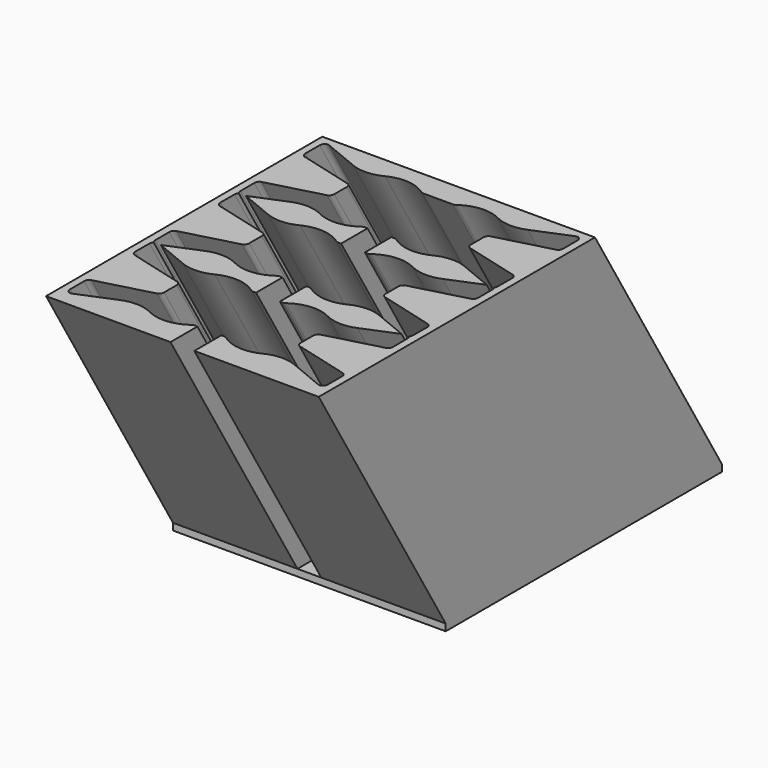
from build123d import *

# Parameters (mm, degrees)
F1_DEPTH  = 88.9
F3_W      = 40.64
F3_H      = 44.1143267043
F4_DEPTH  = 12.7
F9_ANGLE  = -59
F11_W     = 127.9208920896
F11_H     = 131.2496848404
F11_W_2   = 76.2
F11_H_2   = 39.37
F12_DEPTH = 76.2
F14_DEPTH = 1.016


with BuildPart() as f1:
    # F0 (on Front) → F1 (new body)
    with BuildSketch(Plane.XZ):
        with BuildLine():
            Line((-2.2330590469, 18.2673970938), (-1.778, 18.2673970938))
            Line((-1.778, 18.2673970938), (-1.778, 22.4996029062))
            Line((-1.778, 22.4996029062), (-2.2330590469, 22.4996029062))
            ThreePointArc((-2.2330590469, 22.4996029062), (-2.4055915324, 22.4757146321), (-2.5651429052, 22.4058471312))
            ThreePointArc((-2.5651429052, 22.4058471312), (-5.4252105459, 21.4850287563), (-8.3884412084, 21.9821780602))
            ThreePointArc((-8.3884412084, 21.9821780602), (-10.6860377447, 22.4927612394), (-13.0117790963, 22.1314134961))
            Line((-13.0117790963, 22.1314134961), (-17.9445793555, 20.3835))
            Line((-17.9445793555, 20.3835), (-13.0117790963, 18.6355865039))
            ThreePointArc((-13.0117790963, 18.6355865039), (-10.6860377447, 18.2742387606), (-8.3884412084, 18.7848219398))
            ThreePointArc((-8.3884412084, 18.7848219398), (-5.4252105459, 19.2819712437), (-2.5651429052, 18.3611528688))
            ThreePointArc((-2.5651429052, 18.3611528688), (-2.4055915324, 18.2912853679), (-2.2330590469, 18.2673970938))
        make_face()
    extrude(amount=F1_DEPTH)


with BuildPart() as f1b:
    # F0 (on Front) → F1, piece 2 (new body)
    with BuildSketch(Plane.XZ):
        with BuildLine():
            Line((13.0117790963, 18.6355865039), (17.9445793555, 20.3835))
            Line((17.9445793555, 20.3835), (13.0117790963, 22.1314134961))
            ThreePointArc((13.0117790963, 22.1314134961), (10.6860377447, 22.4927612394), (8.3884412084, 21.9821780602))
            ThreePointArc((8.3884412084, 21.9821780602), (5.4252105459, 21.4850287563), (2.5651429052, 22.4058471312))
            ThreePointArc((2.5651429052, 22.4058471312), (2.4055915324, 22.4757146321), (2.2330590469, 22.4996029062))
            Line((2.2330590469, 22.4996029062), (1.778, 22.4996029062))
            Line((1.778, 22.4996029062), (1.778, 18.2673970938))
            Line((1.778, 18.2673970938), (2.2330590469, 18.2673970938))
            ThreePointArc((2.2330590469, 18.2673970938), (2.4055915324, 18.2912853679), (2.5651429052, 18.3611528688))
            ThreePointArc((2.5651429052, 18.3611528688), (5.4252105459, 19.2819712437), (8.3884412084, 18.7848219398))
            ThreePointArc((8.3884412084, 18.7848219398), (10.6860377447, 18.2742387606), (13.0117790963, 18.6355865039))
        make_face()
    extrude(amount=F1_DEPTH)


with BuildPart() as f1c:
    # F0 (on Front) → F1, piece 3 (new body)
    with BuildSketch(Plane.XZ):
        with BuildLine():
            Line((13.0117790963, 5.0465865039), (17.9445793555, 6.7945))
            Line((17.9445793555, 6.7945), (13.0117790963, 8.5424134961))
            ThreePointArc((13.0117790963, 8.5424134961), (10.6860377447, 8.9037612394), (8.3884412084, 8.3931780602))
            ThreePointArc((8.3884412084, 8.3931780602), (5.4252105459, 7.8960287563), (2.5651429052, 8.8168471312))
            ThreePointArc((2.5651429052, 8.8168471312), (2.4055915324, 8.8867146321), (2.2330590469, 8.9106029062))
            Line((2.2330590469, 8.9106029062), (1.778, 8.9106029062))
            Line((1.778, 8.9106029062), (1.778, 4.6783970938))
            Line((1.778, 4.6783970938), (2.2330590469, 4.6783970938))
            ThreePointArc((2.2330590469, 4.6783970938), (2.4055915324, 4.7022853679), (2.5651429052, 4.7721528688))
            ThreePointArc((2.5651429052, 4.7721528688), (5.4252105459, 5.6929712437), (8.3884412084, 5.1958219398))
            ThreePointArc((8.3884412084, 5.1958219398), (10.6860377447, 4.6852387606), (13.0117790963, 5.0465865039))
        make_face()
    extrude(amount=F1_DEPTH)


with BuildPart() as f1d:
    # F0 (on Front) → F1, piece 4 (new body)
    with BuildSketch(Plane.XZ):
        with BuildLine():
            Line((-2.2330590469, 4.6783970938), (-1.778, 4.6783970938))
            Line((-1.778, 4.6783970938), (-1.778, 8.9106029062))
            Line((-1.778, 8.9106029062), (-2.2330590469, 8.9106029062))
            ThreePointArc((-2.2330590469, 8.9106029062), (-2.4055915324, 8.8867146321), (-2.5651429052, 8.8168471312))
            ThreePointArc((-2.5651429052, 8.8168471312), (-5.4252105459, 7.8960287563), (-8.3884412084, 8.3931780602))
            ThreePointArc((-8.3884412084, 8.3931780602), (-10.6860377447, 8.9037612394), (-13.0117790963, 8.5424134961))
            Line((-13.0117790963, 8.5424134961), (-17.9445793555, 6.7945))
            Line((-17.9445793555, 6.7945), (-13.0117790963, 5.0465865039))
            ThreePointArc((-13.0117790963, 5.0465865039), (-10.6860377447, 4.6852387606), (-8.3884412084, 5.1958219398))
            ThreePointArc((-8.3884412084, 5.1958219398), (-5.4252105459, 5.6929712437), (-2.5651429052, 4.7721528688))
            ThreePointArc((-2.5651429052, 4.7721528688), (-2.4055915324, 4.7022853679), (-2.2330590469, 4.6783970938))
        make_face()
    extrude(amount=F1_DEPTH)


with BuildPart() as f1e:
    # F0 (on Front) → F1, piece 5 (new body)
    with BuildSketch(Plane.XZ):
        with BuildLine():
            ThreePointArc((10.6693075207, 1.6245687681), (10.3142300694, 1.4013840597), (10.1757328957, 1.0055179921))
            Line((10.1757328957, 1.0055179921), (10.1757328957, 0))
            Line((10.1757328957, 0), (10.1757328957, -1.0055179921))
            ThreePointArc((10.1757328957, -1.0055179921), (10.3142300694, -1.4013840597), (10.6693075207, -1.6245687681))
            Line((10.6693075207, -1.6245687681), (18.7232144628, -3.4645257695))
            ThreePointArc((18.7232144628, -3.4645257695), (19.0794060399, -3.6891118844), (19.2167789926, -4.0871571512))
            Line((19.2167789926, -4.0871571512), (19.2040435859, -6.3456730598))
            ThreePointArc((19.2040435859, -6.3456730598), (18.9340250914, -6.8617277779), (18.3569658643, -6.9406271299))
            Line((18.3569658643, -6.9406271299), (13.0117790963, -5.0465865039))
            ThreePointArc((13.0117790963, -5.0465865039), (10.6860377447, -4.6852387606), (8.3884412084, -5.1958219398))
            ThreePointArc((8.3884412084, -5.1958219398), (5.4252105459, -5.6929712437), (2.5651429052, -4.7721528688))
            ThreePointArc((2.5651429052, -4.7721528688), (2.4055915324, -4.7022853679), (2.2330590469, -4.6783970938))
            Line((2.2330590469, -4.6783970938), (1.778, -4.6783970938))
            Line((1.778, -4.6783970938), (1.778, -8.9796995744))
            Line((1.778, -8.9796995744), (20.32, -8.9796995744))
            Line((20.32, -8.9796995744), (20.32, 35.1346271299))
            Line((20.32, 35.1346271299), (-20.32, 35.1346271299))
            Line((-20.32, 35.1346271299), (-20.32, -8.9796995744))
            Line((-20.32, -8.9796995744), (-1.778, -8.9796995744))
            Line((-1.778, -8.9796995744), (-1.778, -4.6783970938))
            Line((-1.778, -4.6783970938), (-2.2330590469, -4.6783970938))
            ThreePointArc((-2.2330590469, -4.6783970938), (-2.4055915324, -4.7022853679), (-2.5651429052, -4.7721528688))
            ThreePointArc((-2.5651429052, -4.7721528688), (-5.4252105459, -5.6929712437), (-8.3884412084, -5.1958219398))
            ThreePointArc((-8.3884412084, -5.1958219398), (-10.6860377447, -4.6852387606), (-13.0117790963, -5.0465865039))
            Line((-13.0117790963, -5.0465865039), (-18.3569658643, -6.9406271299))
            ThreePointArc((-18.3569658643, -6.9406271299), (-18.9340250914, -6.8617277779), (-19.2040435859, -6.3456730598))
            Line((-19.2040435859, -6.3456730598), (-19.2167789926, -4.0871571512))
            ThreePointArc((-19.2167789926, -4.0871571512), (-19.0794060399, -3.6891118844), (-18.7232144628, -3.4645257695))
            Line((-18.7232144628, -3.4645257695), (-10.6693075207, -1.6245687681))
            ThreePointArc((-10.6693075207, -1.6245687681), (-10.3142300694, -1.4013840597), (-10.1757328957, -1.0055179921))
            Line((-10.1757328957, -1.0055179921), (-10.1757328957, 0))
            Line((-10.1757328957, 0), (-10.1757328957, 1.0055179921))
            ThreePointArc((-10.1757328957, 1.0055179921), (-10.3142300694, 1.4013840597), (-10.6693075207, 1.6245687681))
            Line((-10.6693075207, 1.6245687681), (-18.7232144628, 3.4645257695))
            ThreePointArc((-18.7232144628, 3.4645257695), (-19.0794060399, 3.6891118844), (-19.2167789926, 4.0871571512))
            Line((-19.2167789926, 4.0871571512), (-19.2040435859, 6.3456730598))
            ThreePointArc((-19.2040435859, 6.3456730598), (-19.1540971232, 6.5889713128), (-19.0146458853, 6.7945))
            ThreePointArc((-19.0146458853, 6.7945), (-19.1540971232, 7.0000286872), (-19.2040435859, 7.2433269402))
            Line((-19.2040435859, 7.2433269402), (-19.2167789926, 9.5018428488))
            ThreePointArc((-19.2167789926, 9.5018428488), (-19.0794060399, 9.8998881156), (-18.7232144628, 10.1244742305))
            Line((-18.7232144628, 10.1244742305), (-10.6693075207, 11.9644312319))
            ThreePointArc((-10.6693075207, 11.9644312319), (-10.3142300694, 12.1876159403), (-10.1757328957, 12.5834820079))
            Line((-10.1757328957, 12.5834820079), (-10.1757328957, 13.589))
            Line((-10.1757328957, 13.589), (-10.1757328957, 14.5945179921))
            ThreePointArc((-10.1757328957, 14.5945179921), (-10.3142300694, 14.9903840597), (-10.6693075207, 15.2135687681))
            Line((-10.6693075207, 15.2135687681), (-18.7232144628, 17.0535257695))
            ThreePointArc((-18.7232144628, 17.0535257695), (-19.0794060399, 17.2781118844), (-19.2167789926, 17.6761571512))
            Line((-19.2167789926, 17.6761571512), (-19.2040435859, 19.9346730598))
            ThreePointArc((-19.2040435859, 19.9346730598), (-19.1540971232, 20.1779713128), (-19.0146458853, 20.3835))
            ThreePointArc((-19.0146458853, 20.3835), (-19.1540971232, 20.5890286872), (-19.2040435859, 20.8323269402))
            Line((-19.2040435859, 20.8323269402), (-19.2167789926, 23.0908428488))
            ThreePointArc((-19.2167789926, 23.0908428488), (-19.0794060399, 23.4888881156), (-18.7232144628, 23.7134742305))
            Line((-18.7232144628, 23.7134742305), (-10.6693075207, 25.5534312319))
            ThreePointArc((-10.6693075207, 25.5534312319), (-10.3142300694, 25.7766159403), (-10.1757328957, 26.1724820079))
            Line((-10.1757328957, 26.1724820079), (-10.1757328957, 27.178))
            Line((-10.1757328957, 27.178), (-10.1757328957, 28.1835179921))
            ThreePointArc((-10.1757328957, 28.1835179921), (-10.3142300694, 28.5793840597), (-10.6693075207, 28.8025687681))
            Line((-10.6693075207, 28.8025687681), (-18.7232144628, 30.6425257695))
            ThreePointArc((-18.7232144628, 30.6425257695), (-19.0794060399, 30.8671118844), (-19.2167789926, 31.2651571512))
            Line((-19.2167789926, 31.2651571512), (-19.2040435859, 33.5236730598))
            ThreePointArc((-19.2040435859, 33.5236730598), (-18.9340250914, 34.0397277779), (-18.3569658643, 34.1186271299))
            Line((-18.3569658643, 34.1186271299), (-13.0117790963, 32.2245865039))
            ThreePointArc((-13.0117790963, 32.2245865039), (-10.6860377447, 31.8632387606), (-8.3884412084, 32.3738219398))
            ThreePointArc((-8.3884412084, 32.3738219398), (-5.4252105459, 32.8709712437), (-2.5651429052, 31.9501528688))
            ThreePointArc((-2.5651429052, 31.9501528688), (-2.4055915324, 31.8802853679), (-2.2330590469, 31.8563970938))
            Line((-2.2330590469, 31.8563970938), (0, 31.8563970938))
            Line((0, 31.8563970938), (2.2330590469, 31.8563970938))
            ThreePointArc((2.2330590469, 31.8563970938), (2.4055915324, 31.8802853679), (2.5651429052, 31.9501528688))
            ThreePointArc((2.5651429052, 31.9501528688), (5.4252105459, 32.8709712437), (8.3884412084, 32.3738219398))
            ThreePointArc((8.3884412084, 32.3738219398), (10.6860377447, 31.8632387606), (13.0117790963, 32.2245865039))
            Line((13.0117790963, 32.2245865039), (18.3569658643, 34.1186271299))
            ThreePointArc((18.3569658643, 34.1186271299), (18.9340250914, 34.0397277779), (19.2040435859, 33.5236730598))
            Line((19.2040435859, 33.5236730598), (19.2167789926, 31.2651571512))
            ThreePointArc((19.2167789926, 31.2651571512), (19.0794060399, 30.8671118844), (18.7232144628, 30.6425257695))
            Line((18.7232144628, 30.6425257695), (10.6693075207, 28.8025687681))
            ThreePointArc((10.6693075207, 28.8025687681), (10.3142300694, 28.5793840597), (10.1757328957, 28.1835179921))
            Line((10.1757328957, 28.1835179921), (10.1757328957, 27.178))
            Line((10.1757328957, 27.178), (10.1757328957, 26.1724820079))
            ThreePointArc((10.1757328957, 26.1724820079), (10.3142300694, 25.7766159403), (10.6693075207, 25.5534312319))
            Line((10.6693075207, 25.5534312319), (18.7232144628, 23.7134742305))
            ThreePointArc((18.7232144628, 23.7134742305), (19.0794060399, 23.4888881156), (19.2167789926, 23.0908428488))
            Line((19.2167789926, 23.0908428488), (19.2040435859, 20.8323269402))
            ThreePointArc((19.2040435859, 20.8323269402), (19.1540971232, 20.5890286872), (19.0146458853, 20.3835))
            ThreePointArc((19.0146458853, 20.3835), (19.1540971232, 20.1779713128), (19.2040435859, 19.9346730598))
            Line((19.2040435859, 19.9346730598), (19.2167789926, 17.6761571512))
            ThreePointArc((19.2167789926, 17.6761571512), (19.0794060399, 17.2781118844), (18.7232144628, 17.0535257695))
            Line((18.7232144628, 17.0535257695), (10.6693075207, 15.2135687681))
            ThreePointArc((10.6693075207, 15.2135687681), (10.3142300694, 14.9903840597), (10.1757328957, 14.5945179921))
            Line((10.1757328957, 14.5945179921), (10.1757328957, 13.589))
            Line((10.1757328957, 13.589), (10.1757328957, 12.5834820079))
            ThreePointArc((10.1757328957, 12.5834820079), (10.3142300694, 12.1876159403), (10.6693075207, 11.9644312319))
            Line((10.6693075207, 11.9644312319), (18.7232144628, 10.1244742305))
            ThreePointArc((18.7232144628, 10.1244742305), (19.0794060399, 9.8998881156), (19.2167789926, 9.5018428488))
            Line((19.2167789926, 9.5018428488), (19.2040435859, 7.2433269402))
            ThreePointArc((19.2040435859, 7.2433269402), (19.1540971232, 7.0000286872), (19.0146458853, 6.7945))
            ThreePointArc((19.0146458853, 6.7945), (19.1540971232, 6.5889713128), (19.2040435859, 6.3456730598))
            Line((19.2040435859, 6.3456730598), (19.2167789926, 4.0871571512))
            ThreePointArc((19.2167789926, 4.0871571512), (19.0794060399, 3.6891118844), (18.7232144628, 3.4645257695))
            Line((18.7232144628, 3.4645257695), (10.6693075207, 1.6245687681))
        make_face()
    extrude(amount=F1_DEPTH)


with BuildPart() as f1e_1:
    # F2: moved
    add(f1e.part.moved(Location((0, 25.4, 0))))


with BuildPart() as f1_1:
    # F2: moved
    add(f1.part.moved(Location((0, 25.4, 0))))



with BuildPart() as f1b_1:
    # F2: moved
    add(f1b.part.moved(Location((0, 25.4, 0))))


with BuildPart() as f1c_1:
    # F2: moved
    add(f1c.part.moved(Location((0, 25.4, 0))))


with BuildPart() as f1d_1:
    # F2: moved
    add(f1d.part.moved(Location((0, 25.4, 0))))


with BuildPart() as f1_2:
    add(f1_1.part)

    add(f1b_1.part)  # F4 merges F1b

    add(f1c_1.part)  # F4 merges F1c

    add(f1d_1.part)  # F4 merges F1d

    add(f1e_1.part)  # F4 merges F1e
    # F3 (on face) → F4 (join)
    with BuildSketch(Plane(origin=(0, 25.4, 0), x_dir=(-1, 0, 0), z_dir=(0, 1, 0))):
        with Locations((0, 13.0774637777)):
            Rectangle(F3_W, F3_H)
    extrude(amount=F4_DEPTH)


with BuildPart() as f1_3:
    # F6: moved
    add(f1_2.part.moved(Location((-20.32, -38.1, -13.0774637777))))


with BuildPart() as f1_4:
    # F7: moved
    add(f1_3.part.moved(Location((0, 38.1, 0))))


with BuildPart() as f1_5:
    # F9: moved
    add(f1_4.part.rotate(Axis((15.9912854433, 0, 0), (1, 0, 0)), F9_ANGLE))

    # F11 (on face) → F12 (cut)
    with BuildSketch(Plane.YZ):
        with Locations((-14.2227876931, 13.1267439574)):
            Rectangle(F11_W, F11_H)
        with Locations((-13.5115969285, 23.3848446437)):
            Rectangle(F11_W_2, F11_H_2, mode=Mode.SUBTRACT)
    extrude(amount=-F12_DEPTH, mode=Mode.SUBTRACT)

    # F13 (on face) → F14 (join)
    with BuildSketch(Plane(origin=(0, 0, 3.6998446437), x_dir=(1, 0, 0), z_dir=(0, 0, -1))):
        with BuildLine():
            Line((-22.098, 27.9557143574), (-40.64, 27.9557143574))
            Line((-40.64, 27.9557143574), (-40.64, -23.5095324715))
            Line((-40.64, -23.5095324715), (0, -23.5095324715))
            Line((0, -23.5095324715), (0, 27.9557143574))
            Line((0, 27.9557143574), (-18.542, 27.9557143574))
            Line((-18.542, 27.9557143574), (-18.542, 22.9376712319))
            Line((-18.542, 22.9376712319), (-18.0869409531, 22.9376712319))
            add(Edge.make_bspline(
                [(-17.7548570948, 23.0470498503), (-17.9076641962, 22.9376712319), (-18.0869409531, 22.9376712319)],
                knots=[5.7328574513, 5.7328574513, 5.7328574513, 6.2831853072, 6.2831853072, 6.2831853072], degree=2, weights=[1, 0.9623806706, 1]))
            add(Edge.make_bspline(
                [(-17.7548570948, 23.0470498503), (-14.9528732156, 25.0526969869), (-11.9315587916, 23.5413163379)],
                knots=[2.5912647978, 2.5912647978, 2.5912647978, 3.5466681465, 3.5466681465, 3.5466681465], degree=2, weights=[1, 0.8880538981, 1]))
            add(Edge.make_bspline(
                [(-7.3082209037, 23.3672132943), (-9.6490726202, 22.3995267235), (-11.9315587916, 23.5413163379)],
                knots=[5.9426448501, 5.9426448501, 5.9426448501, 6.6882608001, 6.6882608001, 6.6882608001], degree=2, weights=[1, 0.9313082643, 1]))
            Line((-7.3082209037, 23.3672132943), (-1.9630341357, 25.5768643443))
            add(Edge.make_bspline(
                [(-1.9630341357, 25.5768643443), (-1.1209937406, 25.9249560994), (-1.1159564141, 24.8827710563)],
                knots=[2.8010521965, 2.8010521965, 2.8010521965, 4.7067502015, 4.7067502015, 4.7067502015], degree=2, weights=[1, 0.5793633091, 1]))
            Line((-1.1159564141, 24.8827710563), (-1.1032210074, 22.2479109692))
            add(Edge.make_bspline(
                [(-1.1032210074, 22.2479109692), (-1.1003496092, 21.6538402352), (-1.5967855372, 21.5215284052)],
                knots=[4.7067502015, 4.7067502015, 4.7067502015, 6.0585845898, 6.0585845898, 6.0585845898], degree=2, weights=[1, 0.7801334707, 1]))
            Line((-1.5967855372, 21.5215284052), (-9.6506924793, 19.3749731179))
            add(Edge.make_bspline(
                [(-10.1442671043, 18.652767808), (-10.1442671043, 19.2434238924), (-9.6506924793, 19.3749731179)],
                knots=[1.5707963268, 1.5707963268, 1.5707963268, 2.9169919362, 2.9169919362, 2.9169919362], degree=2, weights=[1, 0.7818942147, 1]))
            Line((-10.1442671043, 18.652767808), (-10.1442671043, 16.3066260658))
            add(Edge.make_bspline(
                [(-9.6506924793, 15.5844207559), (-10.1442671043, 15.7159699815), (-10.1442671043, 16.3066260658)],
                knots=[0.2246007174, 0.2246007174, 0.2246007174, 1.5707963268, 1.5707963268, 1.5707963268], degree=2, weights=[1, 0.7818942147, 1]))
            Line((-9.6506924793, 15.5844207559), (-1.5967855372, 13.4378654686))
            add(Edge.make_bspline(
                [(-1.5967855372, 13.4378654686), (-1.1003496092, 13.3055536387), (-1.1032210074, 12.7114829047)],
                knots=[3.366193371, 3.366193371, 3.366193371, 4.7180277592, 4.7180277592, 4.7180277592], degree=2, weights=[1, 0.7801334707, 1]))
            Line((-1.1032210074, 12.7114829047), (-1.1159564141, 10.0766228175))
            add(Edge.make_bspline(
                [(-1.1159564141, 10.0766228175), (-1.1174436424, 9.7689264496), (-1.3053541147, 9.5530063195)],
                knots=[4.7180277592, 4.7180277592, 4.7180277592, 5.5053764673, 5.5053764673, 5.5053764673], degree=2, weights=[1, 0.9235058726, 1]))
            add(Edge.make_bspline(
                [(-1.3053541147, 9.5530063195), (-1.1174436424, 9.3370861895), (-1.1159564141, 9.0293898216)],
                knots=[3.9194014935, 3.9194014935, 3.9194014935, 4.7067502015, 4.7067502015, 4.7067502015], degree=2, weights=[1, 0.9235058726, 1]))
            Line((-1.1159564141, 9.0293898216), (-1.1032210074, 6.3945297344))
            add(Edge.make_bspline(
                [(-1.1032210074, 6.3945297344), (-1.1003496092, 5.8004590004), (-1.5967855372, 5.6681471704)],
                knots=[4.7067502015, 4.7067502015, 4.7067502015, 6.0585845898, 6.0585845898, 6.0585845898], degree=2, weights=[1, 0.7801334707, 1]))
            Line((-1.5967855372, 5.6681471704), (-9.6506924793, 3.5215918832))
            add(Edge.make_bspline(
                [(-10.1442671043, 2.7993865733), (-10.1442671043, 3.3900426576), (-9.6506924793, 3.5215918832)],
                knots=[1.5707963268, 1.5707963268, 1.5707963268, 2.9169919362, 2.9169919362, 2.9169919362], degree=2, weights=[1, 0.7818942147, 1]))
            Line((-10.1442671043, 2.7993865733), (-10.1442671043, 0.4532448311))
            add(Edge.make_bspline(
                [(-9.6506924793, -0.2689604788), (-10.1442671043, -0.1374112533), (-10.1442671043, 0.4532448311)],
                knots=[0.2246007174, 0.2246007174, 0.2246007174, 1.5707963268, 1.5707963268, 1.5707963268], degree=2, weights=[1, 0.7818942147, 1]))
            Line((-9.6506924793, -0.2689604788), (-1.5967855372, -2.4155157661))
            add(Edge.make_bspline(
                [(-1.5967855372, -2.4155157661), (-1.1003496092, -2.5478275961), (-1.1032210074, -3.1418983301)],
                knots=[3.366193371, 3.366193371, 3.366193371, 4.7180277592, 4.7180277592, 4.7180277592], degree=2, weights=[1, 0.7801334707, 1]))
            Line((-1.1032210074, -3.1418983301), (-1.1159564141, -5.7767584173))
            add(Edge.make_bspline(
                [(-1.1159564141, -5.7767584173), (-1.1174436424, -6.0844547852), (-1.3053541147, -6.3003749152)],
                knots=[4.7180277592, 4.7180277592, 4.7180277592, 5.5053764673, 5.5053764673, 5.5053764673], degree=2, weights=[1, 0.9235058726, 1]))
            add(Edge.make_bspline(
                [(-1.3053541147, -6.3003749152), (-1.1174436424, -6.5162950453), (-1.1159564141, -6.8239914132)],
                knots=[3.9194014935, 3.9194014935, 3.9194014935, 4.7067502015, 4.7067502015, 4.7067502015], degree=2, weights=[1, 0.9235058726, 1]))
            Line((-1.1159564141, -6.8239914132), (-1.1032210074, -9.4588515004))
            add(Edge.make_bspline(
                [(-1.1032210074, -9.4588515004), (-1.1003496092, -10.0529222343), (-1.5967855372, -10.1852340643)],
                knots=[4.7067502015, 4.7067502015, 4.7067502015, 6.0585845898, 6.0585845898, 6.0585845898], degree=2, weights=[1, 0.7801334707, 1]))
            Line((-1.5967855372, -10.1852340643), (-9.6506924793, -12.3317893516))
            add(Edge.make_bspline(
                [(-10.1442671043, -13.0539946615), (-10.1442671043, -12.4633385772), (-9.6506924793, -12.3317893516)],
                knots=[1.5707963268, 1.5707963268, 1.5707963268, 2.9169919362, 2.9169919362, 2.9169919362], degree=2, weights=[1, 0.7818942147, 1]))
            Line((-10.1442671043, -13.0539946615), (-10.1442671043, -15.4001364037))
            add(Edge.make_bspline(
                [(-9.6506924793, -16.1223417136), (-10.1442671043, -15.990792488), (-10.1442671043, -15.4001364037)],
                knots=[0.2246007174, 0.2246007174, 0.2246007174, 1.5707963268, 1.5707963268, 1.5707963268], degree=2, weights=[1, 0.7818942147, 1]))
            Line((-9.6506924793, -16.1223417136), (-1.5967855372, -18.2688970009))
            add(Edge.make_bspline(
                [(-1.5967855372, -18.2688970009), (-1.1003496092, -18.4012088309), (-1.1032210074, -18.9952795648)],
                knots=[3.366193371, 3.366193371, 3.366193371, 4.7180277592, 4.7180277592, 4.7180277592], degree=2, weights=[1, 0.7801334707, 1]))
            Line((-1.1032210074, -18.9952795648), (-1.1159564141, -21.630139652))
            add(Edge.make_bspline(
                [(-1.1159564141, -21.630139652), (-1.1209937406, -22.672324695), (-1.9630341357, -22.32423294)],
                knots=[4.7180277592, 4.7180277592, 4.7180277592, 6.6237257642, 6.6237257642, 6.6237257642], degree=2, weights=[1, 0.5793633091, 1]))
            Line((-1.9630341357, -22.32423294), (-7.3082209037, -20.11458189))
            add(Edge.make_bspline(
                [(-11.9315587916, -20.2886849336), (-9.6490726202, -19.1468953192), (-7.3082209037, -20.11458189)],
                knots=[2.7365171607, 2.7365171607, 2.7365171607, 3.4821331107, 3.4821331107, 3.4821331107], degree=2, weights=[1, 0.9313082643, 1]))
            add(Edge.make_bspline(
                [(-11.9315587916, -20.2886849336), (-14.9528732156, -21.8000655826), (-17.7548570948, -19.7944184459)],
                knots=[5.8781098143, 5.8781098143, 5.8781098143, 6.833513163, 6.833513163, 6.833513163], degree=2, weights=[1, 0.8880538981, 1]))
            add(Edge.make_bspline(
                [(-18.0869409531, -19.6850398276), (-17.9076641962, -19.6850398276), (-17.7548570948, -19.7944184459)],
                knots=[3.1415926536, 3.1415926536, 3.1415926536, 3.6919205094, 3.6919205094, 3.6919205094], degree=2, weights=[1, 0.9623806706, 1]))
            Line((-18.0869409531, -19.6850398276), (-22.5530590469, -19.6850398276))
            add(Edge.make_bspline(
                [(-22.8851429052, -19.7944184459), (-22.7323358038, -19.6850398276), (-22.5530590469, -19.6850398276)],
                knots=[2.5912647978, 2.5912647978, 2.5912647978, 3.1415926536, 3.1415926536, 3.1415926536], degree=2, weights=[1, 0.9623806706, 1]))
            add(Edge.make_bspline(
                [(-22.8851429052, -19.7944184459), (-25.6871267844, -21.8000655826), (-28.7084412084, -20.2886849336)],
                knots=[5.7328574513, 5.7328574513, 5.7328574513, 6.6882608001, 6.6882608001, 6.6882608001], degree=2, weights=[1, 0.8880538981, 1]))
            add(Edge.make_bspline(
                [(-33.3317790963, -20.11458189), (-30.9909273798, -19.1468953192), (-28.7084412084, -20.2886849336)],
                knots=[2.8010521965, 2.8010521965, 2.8010521965, 3.5466681465, 3.5466681465, 3.5466681465], degree=2, weights=[1, 0.9313082643, 1]))
            Line((-33.3317790963, -20.11458189), (-38.6769658643, -22.32423294))
            add(Edge.make_bspline(
                [(-38.6769658643, -22.32423294), (-39.5190062594, -22.672324695), (-39.5240435859, -21.630139652)],
                knots=[5.9426448501, 5.9426448501, 5.9426448501, 7.8483428551, 7.8483428551, 7.8483428551], degree=2, weights=[1, 0.5793633091, 1]))
            Line((-39.5240435859, -21.630139652), (-39.5367789926, -18.9952795648))
            add(Edge.make_bspline(
                [(-39.5367789926, -18.9952795648), (-39.5396503908, -18.4012088309), (-39.0432144628, -18.2688970009)],
                knots=[1.5651575479, 1.5651575479, 1.5651575479, 2.9169919362, 2.9169919362, 2.9169919362], degree=2, weights=[1, 0.7801334707, 1]))
            Line((-39.0432144628, -18.2688970009), (-30.9893075207, -16.1223417136))
            add(Edge.make_bspline(
                [(-30.4957328957, -15.4001364037), (-30.4957328957, -15.990792488), (-30.9893075207, -16.1223417136)],
                knots=[4.7123889804, 4.7123889804, 4.7123889804, 6.0585845898, 6.0585845898, 6.0585845898], degree=2, weights=[1, 0.7818942147, 1]))
            Line((-30.4957328957, -15.4001364037), (-30.4957328957, -13.0539946615))
            add(Edge.make_bspline(
                [(-30.9893075207, -12.3317893516), (-30.4957328957, -12.4633385772), (-30.4957328957, -13.0539946615)],
                knots=[3.366193371, 3.366193371, 3.366193371, 4.7123889804, 4.7123889804, 4.7123889804], degree=2, weights=[1, 0.7818942147, 1]))
            Line((-30.9893075207, -12.3317893516), (-39.0432144628, -10.1852340643))
            add(Edge.make_bspline(
                [(-39.0432144628, -10.1852340643), (-39.5396503908, -10.0529222343), (-39.5367789926, -9.4588515004)],
                knots=[0.2246007174, 0.2246007174, 0.2246007174, 1.5764351057, 1.5764351057, 1.5764351057], degree=2, weights=[1, 0.7801334707, 1]))
            Line((-39.5367789926, -9.4588515004), (-39.5240435859, -6.8239914132))
            add(Edge.make_bspline(
                [(-39.5240435859, -6.8239914132), (-39.5225563576, -6.5162950453), (-39.3346458853, -6.3003749152)],
                knots=[1.5764351057, 1.5764351057, 1.5764351057, 2.3637838137, 2.3637838137, 2.3637838137], degree=2, weights=[1, 0.9235058726, 1]))
            add(Edge.make_bspline(
                [(-39.3346458853, -6.3003749152), (-39.5225563576, -6.0844547852), (-39.5240435859, -5.7767584173)],
                knots=[0.7778088399, 0.7778088399, 0.7778088399, 1.5651575479, 1.5651575479, 1.5651575479], degree=2, weights=[1, 0.9235058726, 1]))
            Line((-39.5240435859, -5.7767584173), (-39.5367789926, -3.1418983301))
            add(Edge.make_bspline(
                [(-39.5367789926, -3.1418983301), (-39.5396503908, -2.5478275961), (-39.0432144628, -2.4155157661)],
                knots=[1.5651575479, 1.5651575479, 1.5651575479, 2.9169919362, 2.9169919362, 2.9169919362], degree=2, weights=[1, 0.7801334707, 1]))
            Line((-39.0432144628, -2.4155157661), (-30.9893075207, -0.2689604788))
            add(Edge.make_bspline(
                [(-30.4957328957, 0.4532448311), (-30.4957328957, -0.1374112533), (-30.9893075207, -0.2689604788)],
                knots=[4.7123889804, 4.7123889804, 4.7123889804, 6.0585845898, 6.0585845898, 6.0585845898], degree=2, weights=[1, 0.7818942147, 1]))
            Line((-30.4957328957, 0.4532448311), (-30.4957328957, 2.7993865733))
            add(Edge.make_bspline(
                [(-30.9893075207, 3.5215918832), (-30.4957328957, 3.3900426576), (-30.4957328957, 2.7993865733)],
                knots=[3.366193371, 3.366193371, 3.366193371, 4.7123889804, 4.7123889804, 4.7123889804], degree=2, weights=[1, 0.7818942147, 1]))
            Line((-30.9893075207, 3.5215918832), (-39.0432144628, 5.6681471704))
            add(Edge.make_bspline(
                [(-39.0432144628, 5.6681471704), (-39.5396503908, 5.8004590004), (-39.5367789926, 6.3945297344)],
                knots=[0.2246007174, 0.2246007174, 0.2246007174, 1.5764351057, 1.5764351057, 1.5764351057], degree=2, weights=[1, 0.7801334707, 1]))
            Line((-39.5367789926, 6.3945297344), (-39.5240435859, 9.0293898216))
            add(Edge.make_bspline(
                [(-39.5240435859, 9.0293898216), (-39.5225563576, 9.3370861895), (-39.3346458853, 9.5530063195)],
                knots=[1.5764351057, 1.5764351057, 1.5764351057, 2.3637838137, 2.3637838137, 2.3637838137], degree=2, weights=[1, 0.9235058726, 1]))
            add(Edge.make_bspline(
                [(-39.3346458853, 9.5530063195), (-39.5225563576, 9.7689264496), (-39.5240435859, 10.0766228175)],
                knots=[0.7778088399, 0.7778088399, 0.7778088399, 1.5651575479, 1.5651575479, 1.5651575479], degree=2, weights=[1, 0.9235058726, 1]))
            Line((-39.5240435859, 10.0766228175), (-39.5367789926, 12.7114829047))
            add(Edge.make_bspline(
                [(-39.5367789926, 12.7114829047), (-39.5396503908, 13.3055536387), (-39.0432144628, 13.4378654686)],
                knots=[1.5651575479, 1.5651575479, 1.5651575479, 2.9169919362, 2.9169919362, 2.9169919362], degree=2, weights=[1, 0.7801334707, 1]))
            Line((-39.0432144628, 13.4378654686), (-30.9893075207, 15.5844207559))
            add(Edge.make_bspline(
                [(-30.4957328957, 16.3066260658), (-30.4957328957, 15.7159699815), (-30.9893075207, 15.5844207559)],
                knots=[4.7123889804, 4.7123889804, 4.7123889804, 6.0585845898, 6.0585845898, 6.0585845898], degree=2, weights=[1, 0.7818942147, 1]))
            Line((-30.4957328957, 16.3066260658), (-30.4957328957, 18.652767808))
            add(Edge.make_bspline(
                [(-30.9893075207, 19.3749731179), (-30.4957328957, 19.2434238924), (-30.4957328957, 18.652767808)],
                knots=[3.366193371, 3.366193371, 3.366193371, 4.7123889804, 4.7123889804, 4.7123889804], degree=2, weights=[1, 0.7818942147, 1]))
            Line((-30.9893075207, 19.3749731179), (-39.0432144628, 21.5215284052))
            add(Edge.make_bspline(
                [(-39.0432144628, 21.5215284052), (-39.5396503908, 21.6538402352), (-39.5367789926, 22.2479109692)],
                knots=[0.2246007174, 0.2246007174, 0.2246007174, 1.5764351057, 1.5764351057, 1.5764351057], degree=2, weights=[1, 0.7801334707, 1]))
            Line((-39.5367789926, 22.2479109692), (-39.5240435859, 24.8827710563))
            add(Edge.make_bspline(
                [(-39.5240435859, 24.8827710563), (-39.5190062594, 25.9249560994), (-38.6769658643, 25.5768643443)],
                knots=[1.5764351057, 1.5764351057, 1.5764351057, 3.4821331107, 3.4821331107, 3.4821331107], degree=2, weights=[1, 0.5793633091, 1]))
            Line((-38.6769658643, 25.5768643443), (-33.3317790963, 23.3672132943))
            add(Edge.make_bspline(
                [(-28.7084412084, 23.5413163379), (-30.9909273798, 22.3995267235), (-33.3317790963, 23.3672132943)],
                knots=[5.8781098143, 5.8781098143, 5.8781098143, 6.6237257642, 6.6237257642, 6.6237257642], degree=2, weights=[1, 0.9313082643, 1]))
            add(Edge.make_bspline(
                [(-28.7084412084, 23.5413163379), (-25.6871267844, 25.0526969869), (-22.8851429052, 23.0470498503)],
                knots=[2.7365171607, 2.7365171607, 2.7365171607, 3.6919205094, 3.6919205094, 3.6919205094], degree=2, weights=[1, 0.8880538981, 1]))
            add(Edge.make_bspline(
                [(-22.5530590469, 22.9376712319), (-22.7323358038, 22.9376712319), (-22.8851429052, 23.0470498503)],
                knots=[0, 0, 0, 0.5503278558, 0.5503278558, 0.5503278558], degree=2, weights=[1, 0.9623806706, 1]))
            Line((-22.5530590469, 22.9376712319), (-22.098, 22.9376712319))
            Line((-22.098, 22.9376712319), (-22.098, 27.9557143574))
        make_face()
        with BuildLine():
            Line((-18.542, 27.9557143574), (-22.098, 27.9557143574))
            Line((-22.098, 27.9557143574), (-22.098, 22.9376712319))
            Line((-22.098, 22.9376712319), (-22.5530590469, 22.9376712319))
            add(Edge.make_bspline(
                [(-22.5530590469, 22.9376712319), (-22.7323358038, 22.9376712319), (-22.8851429052, 23.0470498503)],
                knots=[0, 0, 0, 0.5503278558, 0.5503278558, 0.5503278558], degree=2, weights=[1, 0.9623806706, 1]))
            add(Edge.make_bspline(
                [(-28.7084412084, 23.5413163379), (-25.6871267844, 25.0526969869), (-22.8851429052, 23.0470498503)],
                knots=[2.7365171607, 2.7365171607, 2.7365171607, 3.6919205094, 3.6919205094, 3.6919205094], degree=2, weights=[1, 0.8880538981, 1]))
            add(Edge.make_bspline(
                [(-28.7084412084, 23.5413163379), (-30.9909273798, 22.3995267235), (-33.3317790963, 23.3672132943)],
                knots=[5.8781098143, 5.8781098143, 5.8781098143, 6.6237257642, 6.6237257642, 6.6237257642], degree=2, weights=[1, 0.9313082643, 1]))
            Line((-33.3317790963, 23.3672132943), (-38.6769658643, 25.5768643443))
            add(Edge.make_bspline(
                [(-39.5240435859, 24.8827710563), (-39.5190062594, 25.9249560994), (-38.6769658643, 25.5768643443)],
                knots=[1.5764351057, 1.5764351057, 1.5764351057, 3.4821331107, 3.4821331107, 3.4821331107], degree=2, weights=[1, 0.5793633091, 1]))
            Line((-39.5240435859, 24.8827710563), (-39.5367789926, 22.2479109692))
            add(Edge.make_bspline(
                [(-39.0432144628, 21.5215284052), (-39.5396503908, 21.6538402352), (-39.5367789926, 22.2479109692)],
                knots=[0.2246007174, 0.2246007174, 0.2246007174, 1.5764351057, 1.5764351057, 1.5764351057], degree=2, weights=[1, 0.7801334707, 1]))
            Line((-39.0432144628, 21.5215284052), (-30.9893075207, 19.3749731179))
            add(Edge.make_bspline(
                [(-30.9893075207, 19.3749731179), (-30.4957328957, 19.2434238924), (-30.4957328957, 18.652767808)],
                knots=[3.366193371, 3.366193371, 3.366193371, 4.7123889804, 4.7123889804, 4.7123889804], degree=2, weights=[1, 0.7818942147, 1]))
            Line((-30.4957328957, 18.652767808), (-30.4957328957, 16.3066260658))
            add(Edge.make_bspline(
                [(-30.4957328957, 16.3066260658), (-30.4957328957, 15.7159699815), (-30.9893075207, 15.5844207559)],
                knots=[4.7123889804, 4.7123889804, 4.7123889804, 6.0585845898, 6.0585845898, 6.0585845898], degree=2, weights=[1, 0.7818942147, 1]))
            Line((-30.9893075207, 15.5844207559), (-39.0432144628, 13.4378654686))
            add(Edge.make_bspline(
                [(-39.5367789926, 12.7114829047), (-39.5396503908, 13.3055536387), (-39.0432144628, 13.4378654686)],
                knots=[1.5651575479, 1.5651575479, 1.5651575479, 2.9169919362, 2.9169919362, 2.9169919362], degree=2, weights=[1, 0.7801334707, 1]))
            Line((-39.5367789926, 12.7114829047), (-39.5240435859, 10.0766228175))
            add(Edge.make_bspline(
                [(-39.3346458853, 9.5530063195), (-39.5225563576, 9.7689264496), (-39.5240435859, 10.0766228175)],
                knots=[0.7778088399, 0.7778088399, 0.7778088399, 1.5651575479, 1.5651575479, 1.5651575479], degree=2, weights=[1, 0.9235058726, 1]))
            add(Edge.make_bspline(
                [(-39.5240435859, 9.0293898216), (-39.5225563576, 9.3370861895), (-39.3346458853, 9.5530063195)],
                knots=[1.5764351057, 1.5764351057, 1.5764351057, 2.3637838137, 2.3637838137, 2.3637838137], degree=2, weights=[1, 0.9235058726, 1]))
            Line((-39.5240435859, 9.0293898216), (-39.5367789926, 6.3945297344))
            add(Edge.make_bspline(
                [(-39.0432144628, 5.6681471704), (-39.5396503908, 5.8004590004), (-39.5367789926, 6.3945297344)],
                knots=[0.2246007174, 0.2246007174, 0.2246007174, 1.5764351057, 1.5764351057, 1.5764351057], degree=2, weights=[1, 0.7801334707, 1]))
            Line((-39.0432144628, 5.6681471704), (-30.9893075207, 3.5215918832))
            add(Edge.make_bspline(
                [(-30.9893075207, 3.5215918832), (-30.4957328957, 3.3900426576), (-30.4957328957, 2.7993865733)],
                knots=[3.366193371, 3.366193371, 3.366193371, 4.7123889804, 4.7123889804, 4.7123889804], degree=2, weights=[1, 0.7818942147, 1]))
            Line((-30.4957328957, 2.7993865733), (-30.4957328957, 0.4532448311))
            add(Edge.make_bspline(
                [(-30.4957328957, 0.4532448311), (-30.4957328957, -0.1374112533), (-30.9893075207, -0.2689604788)],
                knots=[4.7123889804, 4.7123889804, 4.7123889804, 6.0585845898, 6.0585845898, 6.0585845898], degree=2, weights=[1, 0.7818942147, 1]))
            Line((-30.9893075207, -0.2689604788), (-39.0432144628, -2.4155157661))
            add(Edge.make_bspline(
                [(-39.5367789926, -3.1418983301), (-39.5396503908, -2.5478275961), (-39.0432144628, -2.4155157661)],
                knots=[1.5651575479, 1.5651575479, 1.5651575479, 2.9169919362, 2.9169919362, 2.9169919362], degree=2, weights=[1, 0.7801334707, 1]))
            Line((-39.5367789926, -3.1418983301), (-39.5240435859, -5.7767584173))
            add(Edge.make_bspline(
                [(-39.3346458853, -6.3003749152), (-39.5225563576, -6.0844547852), (-39.5240435859, -5.7767584173)],
                knots=[0.7778088399, 0.7778088399, 0.7778088399, 1.5651575479, 1.5651575479, 1.5651575479], degree=2, weights=[1, 0.9235058726, 1]))
            add(Edge.make_bspline(
                [(-39.5240435859, -6.8239914132), (-39.5225563576, -6.5162950453), (-39.3346458853, -6.3003749152)],
                knots=[1.5764351057, 1.5764351057, 1.5764351057, 2.3637838137, 2.3637838137, 2.3637838137], degree=2, weights=[1, 0.9235058726, 1]))
            Line((-39.5240435859, -6.8239914132), (-39.5367789926, -9.4588515004))
            add(Edge.make_bspline(
                [(-39.0432144628, -10.1852340643), (-39.5396503908, -10.0529222343), (-39.5367789926, -9.4588515004)],
                knots=[0.2246007174, 0.2246007174, 0.2246007174, 1.5764351057, 1.5764351057, 1.5764351057], degree=2, weights=[1, 0.7801334707, 1]))
            Line((-39.0432144628, -10.1852340643), (-30.9893075207, -12.3317893516))
            add(Edge.make_bspline(
                [(-30.9893075207, -12.3317893516), (-30.4957328957, -12.4633385772), (-30.4957328957, -13.0539946615)],
                knots=[3.366193371, 3.366193371, 3.366193371, 4.7123889804, 4.7123889804, 4.7123889804], degree=2, weights=[1, 0.7818942147, 1]))
            Line((-30.4957328957, -13.0539946615), (-30.4957328957, -15.4001364037))
            add(Edge.make_bspline(
                [(-30.4957328957, -15.4001364037), (-30.4957328957, -15.990792488), (-30.9893075207, -16.1223417136)],
                knots=[4.7123889804, 4.7123889804, 4.7123889804, 6.0585845898, 6.0585845898, 6.0585845898], degree=2, weights=[1, 0.7818942147, 1]))
            Line((-30.9893075207, -16.1223417136), (-39.0432144628, -18.2688970009))
            add(Edge.make_bspline(
                [(-39.5367789926, -18.9952795648), (-39.5396503908, -18.4012088309), (-39.0432144628, -18.2688970009)],
                knots=[1.5651575479, 1.5651575479, 1.5651575479, 2.9169919362, 2.9169919362, 2.9169919362], degree=2, weights=[1, 0.7801334707, 1]))
            Line((-39.5367789926, -18.9952795648), (-39.5240435859, -21.630139652))
            add(Edge.make_bspline(
                [(-38.6769658643, -22.32423294), (-39.5190062594, -22.672324695), (-39.5240435859, -21.630139652)],
                knots=[5.9426448501, 5.9426448501, 5.9426448501, 7.8483428551, 7.8483428551, 7.8483428551], degree=2, weights=[1, 0.5793633091, 1]))
            Line((-38.6769658643, -22.32423294), (-33.3317790963, -20.11458189))
            add(Edge.make_bspline(
                [(-33.3317790963, -20.11458189), (-30.9909273798, -19.1468953192), (-28.7084412084, -20.2886849336)],
                knots=[2.8010521965, 2.8010521965, 2.8010521965, 3.5466681465, 3.5466681465, 3.5466681465], degree=2, weights=[1, 0.9313082643, 1]))
            add(Edge.make_bspline(
                [(-22.8851429052, -19.7944184459), (-25.6871267844, -21.8000655826), (-28.7084412084, -20.2886849336)],
                knots=[5.7328574513, 5.7328574513, 5.7328574513, 6.6882608001, 6.6882608001, 6.6882608001], degree=2, weights=[1, 0.8880538981, 1]))
            add(Edge.make_bspline(
                [(-22.8851429052, -19.7944184459), (-22.7323358038, -19.6850398276), (-22.5530590469, -19.6850398276)],
                knots=[2.5912647978, 2.5912647978, 2.5912647978, 3.1415926536, 3.1415926536, 3.1415926536], degree=2, weights=[1, 0.9623806706, 1]))
            Line((-22.5530590469, -19.6850398276), (-18.0869409531, -19.6850398276))
            add(Edge.make_bspline(
                [(-18.0869409531, -19.6850398276), (-17.9076641962, -19.6850398276), (-17.7548570948, -19.7944184459)],
                knots=[3.1415926536, 3.1415926536, 3.1415926536, 3.6919205094, 3.6919205094, 3.6919205094], degree=2, weights=[1, 0.9623806706, 1]))
            add(Edge.make_bspline(
                [(-11.9315587916, -20.2886849336), (-14.9528732156, -21.8000655826), (-17.7548570948, -19.7944184459)],
                knots=[5.8781098143, 5.8781098143, 5.8781098143, 6.833513163, 6.833513163, 6.833513163], degree=2, weights=[1, 0.8880538981, 1]))
            add(Edge.make_bspline(
                [(-11.9315587916, -20.2886849336), (-9.6490726202, -19.1468953192), (-7.3082209037, -20.11458189)],
                knots=[2.7365171607, 2.7365171607, 2.7365171607, 3.4821331107, 3.4821331107, 3.4821331107], degree=2, weights=[1, 0.9313082643, 1]))
            Line((-7.3082209037, -20.11458189), (-1.9630341357, -22.32423294))
            add(Edge.make_bspline(
                [(-1.1159564141, -21.630139652), (-1.1209937406, -22.672324695), (-1.9630341357, -22.32423294)],
                knots=[4.7180277592, 4.7180277592, 4.7180277592, 6.6237257642, 6.6237257642, 6.6237257642], degree=2, weights=[1, 0.5793633091, 1]))
            Line((-1.1159564141, -21.630139652), (-1.1032210074, -18.9952795648))
            add(Edge.make_bspline(
                [(-1.5967855372, -18.2688970009), (-1.1003496092, -18.4012088309), (-1.1032210074, -18.9952795648)],
                knots=[3.366193371, 3.366193371, 3.366193371, 4.7180277592, 4.7180277592, 4.7180277592], degree=2, weights=[1, 0.7801334707, 1]))
            Line((-1.5967855372, -18.2688970009), (-9.6506924793, -16.1223417136))
            add(Edge.make_bspline(
                [(-9.6506924793, -16.1223417136), (-10.1442671043, -15.990792488), (-10.1442671043, -15.4001364037)],
                knots=[0.2246007174, 0.2246007174, 0.2246007174, 1.5707963268, 1.5707963268, 1.5707963268], degree=2, weights=[1, 0.7818942147, 1]))
            Line((-10.1442671043, -15.4001364037), (-10.1442671043, -13.0539946615))
            add(Edge.make_bspline(
                [(-10.1442671043, -13.0539946615), (-10.1442671043, -12.4633385772), (-9.6506924793, -12.3317893516)],
                knots=[1.5707963268, 1.5707963268, 1.5707963268, 2.9169919362, 2.9169919362, 2.9169919362], degree=2, weights=[1, 0.7818942147, 1]))
            Line((-9.6506924793, -12.3317893516), (-1.5967855372, -10.1852340643))
            add(Edge.make_bspline(
                [(-1.1032210074, -9.4588515004), (-1.1003496092, -10.0529222343), (-1.5967855372, -10.1852340643)],
                knots=[4.7067502015, 4.7067502015, 4.7067502015, 6.0585845898, 6.0585845898, 6.0585845898], degree=2, weights=[1, 0.7801334707, 1]))
            Line((-1.1032210074, -9.4588515004), (-1.1159564141, -6.8239914132))
            add(Edge.make_bspline(
                [(-1.3053541147, -6.3003749152), (-1.1174436424, -6.5162950453), (-1.1159564141, -6.8239914132)],
                knots=[3.9194014935, 3.9194014935, 3.9194014935, 4.7067502015, 4.7067502015, 4.7067502015], degree=2, weights=[1, 0.9235058726, 1]))
            add(Edge.make_bspline(
                [(-1.1159564141, -5.7767584173), (-1.1174436424, -6.0844547852), (-1.3053541147, -6.3003749152)],
                knots=[4.7180277592, 4.7180277592, 4.7180277592, 5.5053764673, 5.5053764673, 5.5053764673], degree=2, weights=[1, 0.9235058726, 1]))
            Line((-1.1159564141, -5.7767584173), (-1.1032210074, -3.1418983301))
            add(Edge.make_bspline(
                [(-1.5967855372, -2.4155157661), (-1.1003496092, -2.5478275961), (-1.1032210074, -3.1418983301)],
                knots=[3.366193371, 3.366193371, 3.366193371, 4.7180277592, 4.7180277592, 4.7180277592], degree=2, weights=[1, 0.7801334707, 1]))
            Line((-1.5967855372, -2.4155157661), (-9.6506924793, -0.2689604788))
            add(Edge.make_bspline(
                [(-9.6506924793, -0.2689604788), (-10.1442671043, -0.1374112533), (-10.1442671043, 0.4532448311)],
                knots=[0.2246007174, 0.2246007174, 0.2246007174, 1.5707963268, 1.5707963268, 1.5707963268], degree=2, weights=[1, 0.7818942147, 1]))
            Line((-10.1442671043, 0.4532448311), (-10.1442671043, 2.7993865733))
            add(Edge.make_bspline(
                [(-10.1442671043, 2.7993865733), (-10.1442671043, 3.3900426576), (-9.6506924793, 3.5215918832)],
                knots=[1.5707963268, 1.5707963268, 1.5707963268, 2.9169919362, 2.9169919362, 2.9169919362], degree=2, weights=[1, 0.7818942147, 1]))
            Line((-9.6506924793, 3.5215918832), (-1.5967855372, 5.6681471704))
            add(Edge.make_bspline(
                [(-1.1032210074, 6.3945297344), (-1.1003496092, 5.8004590004), (-1.5967855372, 5.6681471704)],
                knots=[4.7067502015, 4.7067502015, 4.7067502015, 6.0585845898, 6.0585845898, 6.0585845898], degree=2, weights=[1, 0.7801334707, 1]))
            Line((-1.1032210074, 6.3945297344), (-1.1159564141, 9.0293898216))
            add(Edge.make_bspline(
                [(-1.3053541147, 9.5530063195), (-1.1174436424, 9.3370861895), (-1.1159564141, 9.0293898216)],
                knots=[3.9194014935, 3.9194014935, 3.9194014935, 4.7067502015, 4.7067502015, 4.7067502015], degree=2, weights=[1, 0.9235058726, 1]))
            add(Edge.make_bspline(
                [(-1.1159564141, 10.0766228175), (-1.1174436424, 9.7689264496), (-1.3053541147, 9.5530063195)],
                knots=[4.7180277592, 4.7180277592, 4.7180277592, 5.5053764673, 5.5053764673, 5.5053764673], degree=2, weights=[1, 0.9235058726, 1]))
            Line((-1.1159564141, 10.0766228175), (-1.1032210074, 12.7114829047))
            add(Edge.make_bspline(
                [(-1.5967855372, 13.4378654686), (-1.1003496092, 13.3055536387), (-1.1032210074, 12.7114829047)],
                knots=[3.366193371, 3.366193371, 3.366193371, 4.7180277592, 4.7180277592, 4.7180277592], degree=2, weights=[1, 0.7801334707, 1]))
            Line((-1.5967855372, 13.4378654686), (-9.6506924793, 15.5844207559))
            add(Edge.make_bspline(
                [(-9.6506924793, 15.5844207559), (-10.1442671043, 15.7159699815), (-10.1442671043, 16.3066260658)],
                knots=[0.2246007174, 0.2246007174, 0.2246007174, 1.5707963268, 1.5707963268, 1.5707963268], degree=2, weights=[1, 0.7818942147, 1]))
            Line((-10.1442671043, 16.3066260658), (-10.1442671043, 18.652767808))
            add(Edge.make_bspline(
                [(-10.1442671043, 18.652767808), (-10.1442671043, 19.2434238924), (-9.6506924793, 19.3749731179)],
                knots=[1.5707963268, 1.5707963268, 1.5707963268, 2.9169919362, 2.9169919362, 2.9169919362], degree=2, weights=[1, 0.7818942147, 1]))
            Line((-9.6506924793, 19.3749731179), (-1.5967855372, 21.5215284052))
            add(Edge.make_bspline(
                [(-1.1032210074, 22.2479109692), (-1.1003496092, 21.6538402352), (-1.5967855372, 21.5215284052)],
                knots=[4.7067502015, 4.7067502015, 4.7067502015, 6.0585845898, 6.0585845898, 6.0585845898], degree=2, weights=[1, 0.7801334707, 1]))
            Line((-1.1032210074, 22.2479109692), (-1.1159564141, 24.8827710563))
            add(Edge.make_bspline(
                [(-1.9630341357, 25.5768643443), (-1.1209937406, 25.9249560994), (-1.1159564141, 24.8827710563)],
                knots=[2.8010521965, 2.8010521965, 2.8010521965, 4.7067502015, 4.7067502015, 4.7067502015], degree=2, weights=[1, 0.5793633091, 1]))
            Line((-1.9630341357, 25.5768643443), (-7.3082209037, 23.3672132943))
            add(Edge.make_bspline(
                [(-7.3082209037, 23.3672132943), (-9.6490726202, 22.3995267235), (-11.9315587916, 23.5413163379)],
                knots=[5.9426448501, 5.9426448501, 5.9426448501, 6.6882608001, 6.6882608001, 6.6882608001], degree=2, weights=[1, 0.9313082643, 1]))
            add(Edge.make_bspline(
                [(-17.7548570948, 23.0470498503), (-14.9528732156, 25.0526969869), (-11.9315587916, 23.5413163379)],
                knots=[2.5912647978, 2.5912647978, 2.5912647978, 3.5466681465, 3.5466681465, 3.5466681465], degree=2, weights=[1, 0.8880538981, 1]))
            add(Edge.make_bspline(
                [(-17.7548570948, 23.0470498503), (-17.9076641962, 22.9376712319), (-18.0869409531, 22.9376712319)],
                knots=[5.7328574513, 5.7328574513, 5.7328574513, 6.2831853072, 6.2831853072, 6.2831853072], degree=2, weights=[1, 0.9623806706, 1]))
            Line((-18.0869409531, 22.9376712319), (-18.542, 22.9376712319))
            Line((-18.542, 22.9376712319), (-18.542, 27.9557143574))
        make_face()
    extrude(amount=F14_DEPTH)


solid = f1_5.part
